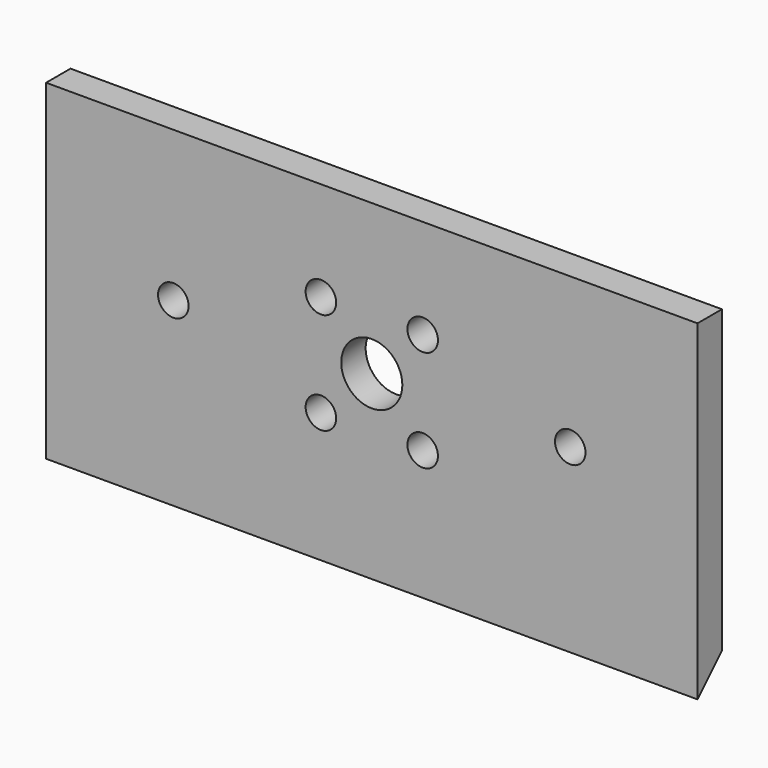
from build123d import *

# Parameters (mm, degrees)
F0_W     = 64
F0_H     = 32.527
F1_DEPTH = 3
F2_SIZE  = 2.99999
F6_D     = 6
F7_D     = 3


# Not quite as in the source:
# - a fillet or chamfer is up to 0.001 mm smaller than in the source, because OpenCascade refuses the exact size


with BuildPart() as f1:
    # F0 (on Front) → F1 (new body)
    with BuildSketch(Plane.XZ):
        with Locations((-32, 16.2635)):
            Rectangle(F0_W, F0_H)
    extrude(amount=F1_DEPTH)

    # F2 (size 3 in the source; OpenCascade refuses exactly that, so slightly less here)
    f2_edges = [f1.edges().sort_by_distance(p)[0] for p in [
        (-32, 0, 0),
    ]]
    chamfer(f2_edges, length=F2_SIZE)

    # F6 (through all)
    with Locations(Plane(origin=(0, 0, 0), x_dir=(-1, 0, 0), z_dir=(0, 1, 0))):
        with Locations((32, 17.7635)):
            Hole(F6_D / 2)

    # F7 (through all)
    with Locations(Plane(origin=(0, 0, 0), x_dir=(-1, 0, 0), z_dir=(0, 1, 0))):
        with Locations((37, 22.7635), (27, 22.7635), (27, 12.7635), (37, 12.7635), (12.5, 17.7635), (51.5, 17.7635)):
            Hole(F7_D / 2)


solid = f1.part
